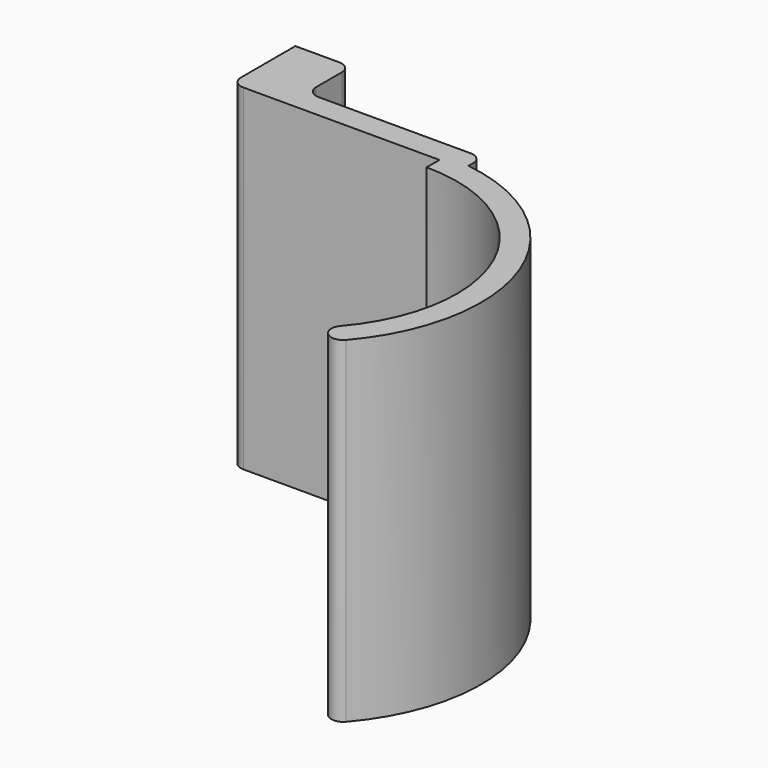
from build123d import *

# Parameters (mm, degrees)
F1_DEPTH = 42
F2_R     = 1.49999
F4_D     = 2.2606
F4_DEPTH = 18.57375
F4_TIP   = 0.6791527577


# Not quite as in the source:
# - a fillet or chamfer is up to 0.001 mm smaller than in the source, because OpenCascade refuses the exact size


with BuildPart() as f1:
    # F0 (on Top) → F1 (new body)
    with BuildSketch(Plane.XY):
        with BuildLine():
            ThreePointArc((0, 19), (17.5537111177, 7.2709852149), (13.4350288425, -13.4350288425))
            Line((13.4350288425, -13.4350288425), (15.5563491861, -15.5563491861))
            ThreePointArc((15.5563491861, -15.5563491861), (20.8531990078, 7.0102846689), (3, 21.7944947177))
            Line((3, 21.7944947177), (3, 24))
            Line((3, 24), (-19, 24))
            Line((-19, 24), (-19, 31))
            Line((-19, 31), (-26, 31))
            Line((-26, 31), (-26, 21))
            Line((-26, 21), (0, 21))
            Line((0, 21), (0, 19))
        make_face()
    extrude(amount=F1_DEPTH)

    # F2 (radius 1.5 in the source; OpenCascade refuses exactly that, so slightly less here)
    f2_edges = [f1.edges().sort_by_distance(p)[0] for p in [
        (13.435029, -13.435029, 21),
        (15.556349, -15.556349, 21),
        (-26, 21, 21),
        (3, 24, 21),
        (-19, 24, 21),
        (-19, 31, 21),
    ]]
    fillet(f2_edges, radius=F2_R)

    # F4
    with Locations(Plane(origin=(-26, 0, 0), x_dir=(0, -1, 0), z_dir=(-1, 0, 0))):
        with Locations((-26, 36), (-26, 6)):
            Hole(F4_D / 2, depth=F4_DEPTH)
            with Locations((0, 0, -(F4_DEPTH + F4_TIP / 2))):  # 118° drill point
                Cone(0, F4_D / 2, F4_TIP, mode=Mode.SUBTRACT)


solid = f1.part
